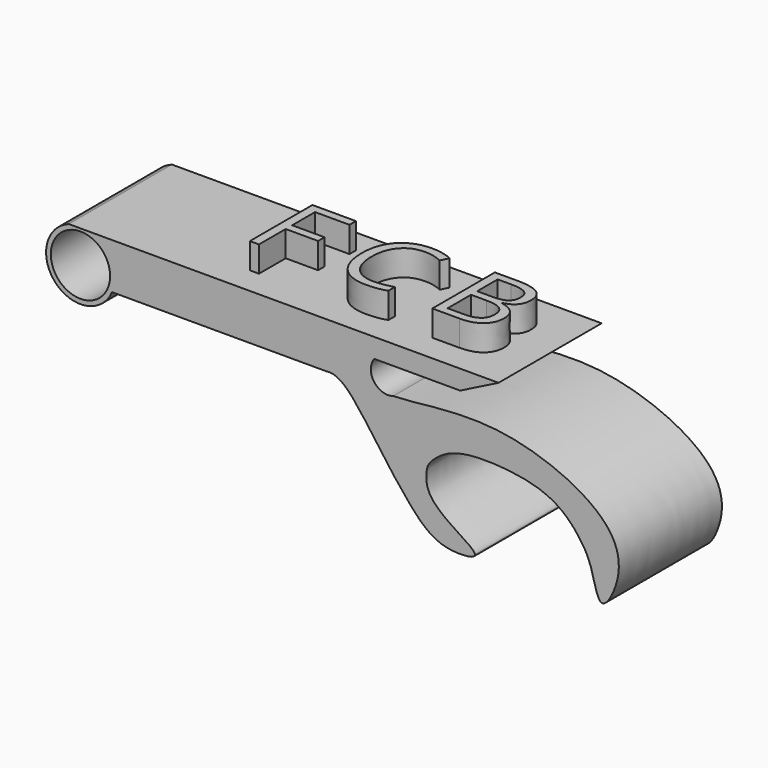
from build123d import *

# Parameters (mm, degrees)
F1_DEPTH     = 15
F2_R         = 3.4504857298
F3_DEPTH     = 25
F4_TEXT_SIZE = 12.7397739561
F5_DEPTH     = 3


# Not quite as in the source:
# - Text() gives the source's letters only with a copy of the font that has no kerning and outlines rounded to 1/6400 em; it was checked with that copy


with BuildPart() as f1:
    # F0 (on Front) → F1 (new body)
    with BuildSketch(Plane.XZ):
        with BuildLine():
            Line((10.7433917001, 0), (0, 0))
            ThreePointArc((0, 0), (-1.5653950383, -6.5081675655), (5.0253296722, -5.3381015517))
            Line((5.0253296722, -5.3381015517), (30.0253296722, -5.3381015517))
            add(Edge.make_bspline(
                [(30.0253296722, -5.3381015517), (31.4228344977, -5.1248271476), (34.0251695987, -8.1417149363), (36.5924299514, -11.9145479357), (39.4705575686, -15.6418587682), (41.7610265019, -18.0615131343), (44.276602554, -19.1709947255), (48.7956554604, -18.8542303242), (43.9548059971, -16.2144652991), (41.5011952592, -13.883907228), (41.5999732876, -11.6891196779), (41.8682852392, -10.762551175), (44.2847169214, -8.5745388648), (49.4748839155, -8.2671849125), (54.8424170385, -9.0635703655), (57.7846219425, -10.8262487138), (59.6737240242, -13.0577236406), (60.9268997827, -15.2723371413), (61.7717592831, -20.2863217061), (64.5822891756, -15.1614769335), (63.2556023033, -9.0582455307), (49.6798591585, -3.3164186654), (40.153587086, -5.3437086706), (37.777474952, -5.3381015517)],
                knots=[0, 0, 0, 0, 0.0502004171, 0.1027848947, 0.1535046064, 0.1956581188, 0.2362941077, 0.2743350111, 0.3195507531, 0.364970538, 0.39694908, 0.4193009789, 0.4590058909, 0.5129972946, 0.5679872999, 0.6108671248, 0.6497113239, 0.6898796551, 0.7321258192, 0.7760858103, 0.8317247898, 0.9198353435, 1, 1, 1, 1], degree=3))
            ThreePointArc((37.777474952, -5.3381015517), (35.523725271, -4.6170337101), (35.5352464031, -2.2507721606))
            Line((35.5352464031, -2.2507721606), (45.5352464031, -2.2507721606))
            Line((45.5352464031, -2.2507721606), (50, 0))
            Line((50, 0), (10.7433917001, 0))
        make_face()
    extrude(amount=F1_DEPTH)

    # F2 (on face) → F3 (cut)
    with BuildSketch(Plane.XZ.offset(15)):
        with Locations((1.3470688679, -3.7663517447)):
            Circle(F2_R)
    extrude(amount=-F3_DEPTH, mode=Mode.SUBTRACT)

    # F4 (on face) → F5 (join)
    with BuildSketch(Plane.XY):
        with Locations((17.2835402191, -11.8370139971)):
            Text('F C B', F4_TEXT_SIZE, font='Open Sans', text_align=(TextAlign.LEFT, TextAlign.BOTTOM))
    extrude(amount=F5_DEPTH)


solid = f1.part
